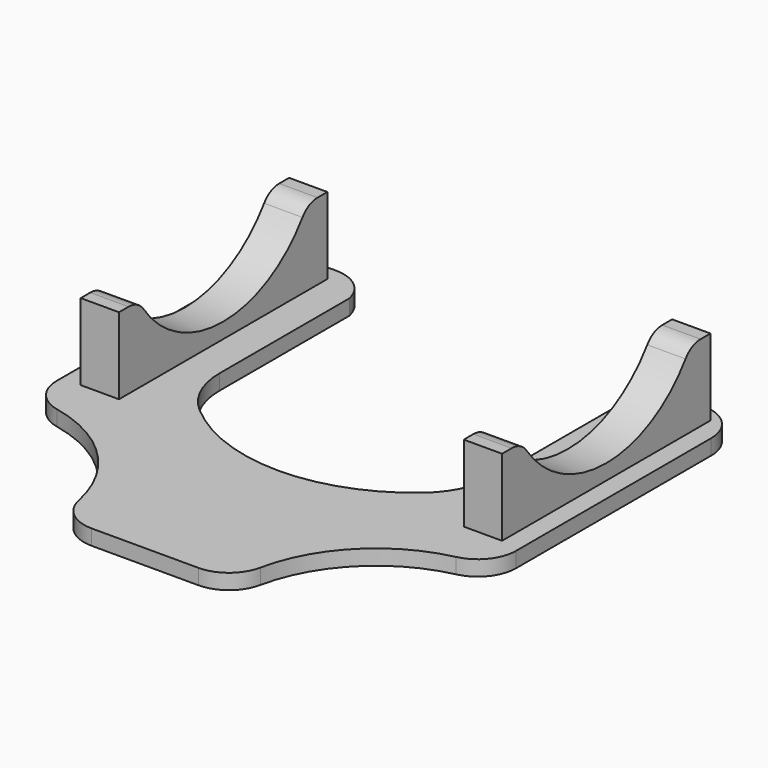
from build123d import *

# Parameters (mm, degrees)
F0_W      = 60
F0_H      = 60
F1_DEPTH  = 2
F2_W      = 5
F2_H      = 34
F3_DEPTH  = 10
F4_R      = 15.85
F5_DEPTH  = 30
F6_R      = 18.5
F7_DEPTH  = 3.5
F8_R      = 5
F10_DEPTH = 4
F11_R     = 10
F12_R     = 3


# Not quite as in the source:
# - a feature names something its author has since deleted; it is built from what else it names


with BuildPart() as f1:
    # F0 (on Top) → F1 (new body)
    with BuildSketch(Plane.XY):
        Rectangle(F0_W, F0_H)
    extrude(amount=-F1_DEPTH)

    # F2 (on face) → F3 (join)
    with BuildSketch(Plane.XY):
        with Locations((-25, 11)):
            Rectangle(F2_W, F2_H)
        with Locations((25, 11)):
            Rectangle(F2_W, F2_H)
    extrude(amount=F3_DEPTH)

    # F4 (on Right) → F5 (cut, symmetric)
    with BuildSketch(Plane.YZ):
        with Locations((10.9725513698, 17.85)):
            Circle(F4_R)
    extrude(amount=F5_DEPTH, both=True, mode=Mode.SUBTRACT)

    # F6 (on Top) → F7 (cut)
    with BuildSketch(Plane.XY):
        with Locations((-29.8706907779, -29.7701153904)):
            Circle(F6_R)
        with Locations((0, 29.9712661654)):
            Circle(F6_R)
        with Locations((30.0718415529, -29.7701153904)):
            Circle(F6_R)
    extrude(amount=-F7_DEPTH, mode=Mode.SUBTRACT)

    # F8
    f8_edges = [f1.edges().sort_by_distance(p)[0] for p in [
        (-30, -11.270567, -1),
        (-11.372119, -30, -1),
        (11.57327, -30, -1),
        (30, -11.270255, -1),
        (30, 30, -1),
        (18.499978, 30, -1),
        (-18.499978, 30, -1),
        (-30, 30, -1),
    ]]
    fillet(f8_edges, radius=F8_R)

    # F9 (on face) → F10 (cut)
    with BuildSketch(Plane.XY):
        with BuildLine():
            Line((18.0813198277, 1.0577162054), (18.0813198277, 26.0577162054))
            ThreePointArc((18.0813198277, 26.0577162054), (0, 11.4712661654), (-18.0813198277, 26.0577162054))
            Line((-18.0813198277, 26.0577162054), (-18.0813198277, 1.0577162054))
            ThreePointArc((-18.0813198277, 1.0577162054), (0, -8.1568370453), (18.0813198277, 1.0577162054))
        make_face()
    extrude(amount=-F10_DEPTH, mode=Mode.SUBTRACT)

    # F11
    f11_edges = [f1.edges().sort_by_distance(p)[0] for p in [
        (-18.08132, 1.057716, -1),
        (18.08132, 1.057716, -1),
    ]]
    fillet(f11_edges, radius=F11_R)

    # F12
    f12_edges = [f1.edges().sort_by_distance(p)[0] for p in [
        (-25, 24.742083, 10),
        (-25, -2.79698, 10),
        (25, 24.742083, 10),
        (25, -2.79698, 10),
    ]]
    fillet(f12_edges, radius=F12_R)


solid = f1.part
